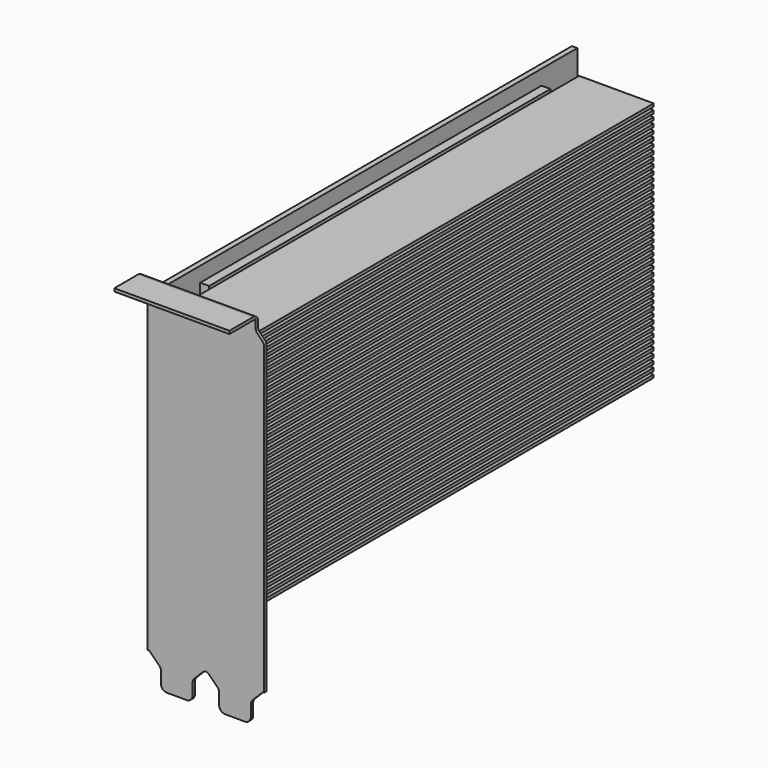
from build123d import *

# Parameters (mm, degrees)
F1_DEPTH    = 1
F2_SIZE     = 4
F0_W        = 38.5976333921
F0_H        = 1
F3_DEPTH    = 12
F4_T1_DEPTH = 1
F4_T3_DEPTH = 48.5976333921
F4_T5_DEPTH = 5.1421356237
F4_T7_DEPTH = 11
F5_W        = 1.8030845018
F5_H        = 92
F6_DEPTH    = 173
F7_W        = 143
F7_H        = 82
F8_DEPTH    = 3
F9_W        = 170
F9_H        = 1
F10_DEPTH   = 25


# Not quite as in the source:
# - a fillet or chamfer that OpenCascade refuses, or shapes differently, is made with other operations: its cross-section is extruded or revolved along the edge and cut away or added


with BuildPart() as f1:
    # F0 (on Front) → F1 (new body)
    with BuildSketch(Plane.XZ):
        Polygon((7.7390509516, 91.1776412405), (10.1390509516, 88.7776412405), (10.1390509516, -14.2223587595), (14.5890509516, -14.2223587595), (14.5890509516, -24.8223587595), (25.1890509516, -24.8223587595), (25.1890509516, -14.2223587595), (29.6390509516, -14.2223587595), (34.0890509516, -14.2223587595), (34.0890509516, -24.8223587595), (44.6890509516, -24.8223587595), (44.6890509516, -14.2223587595), (49.1390509516, -14.2223587595), (49.1390509516, 88.7776412405), (46.3366843437, 91.5800078484), (46.3366843437, 95.1776412405), (7.7390509516, 95.1776412405), align=None)
    extrude(amount=F1_DEPTH)

    # F2
    f2_edges = [f1.edges().sort_by_distance(p)[0] for p in [
        (14.589051, -0.5, -14.222359),
        (25.189051, -0.5, -14.222359),
        (34.089051, -0.5, -14.222359),
        (44.689051, -0.5, -14.222359),
    ]]
    chamfer(f2_edges, length=F2_SIZE)

    # F0 (on Front) → F3 (join)
    with BuildSketch(Plane.XZ):
        with Locations((27.0378676476, 95.6776412405)):
            Rectangle(F0_W, F0_H)
    extrude(amount=F3_DEPTH)

    # F4: fillet of radius 2 on 15 edges, made by hand

    # F4_s2 → F4_t1 (join)
    with BuildSketch(Plane.XZ):
        with BuildLine():
            ThreePointArc((46.3366843437, 92.4084349732), (46.4889252787, 91.6430681084), (46.9224707813, 90.9942214108))
            Line((46.9224707813, 90.9942214108), (46.3366843437, 91.5800078484))
            Line((46.3366843437, 91.5800078484), (46.3366843437, 92.4084349732))
        make_face()
        with BuildLine():
            ThreePointArc((10.1390509516, 87.9492141158), (9.9868100166, 88.7145809805), (9.553264514, 89.3634276781))
            Line((9.553264514, 89.3634276781), (10.1390509516, 88.7776412405))
            Line((10.1390509516, 88.7776412405), (10.1390509516, 87.9492141158))
        make_face()
        with BuildLine():
            ThreePointArc((14.003264514, -17.6365723219), (14.4368100166, -18.2854190195), (14.5890509516, -19.0507858842))
            Line((14.5890509516, -19.0507858842), (14.5890509516, -18.2223587595))
            Line((14.5890509516, -18.2223587595), (14.003264514, -17.6365723219))
        make_face()
        with BuildLine():
            ThreePointArc((25.1890509516, -19.0507858842), (25.3412918866, -18.2854190195), (25.7748373892, -17.6365723219))
            Line((25.7748373892, -17.6365723219), (25.1890509516, -18.2223587595))
            Line((25.1890509516, -18.2223587595), (25.1890509516, -19.0507858842))
        make_face()
        with BuildLine():
            ThreePointArc((28.603264514, -14.8081451971), (29.2521112116, -14.3745996945), (30.0174780763, -14.2223587595))
            Line((30.0174780763, -14.2223587595), (29.1890509516, -14.2223587595))
            Line((29.1890509516, -14.2223587595), (28.603264514, -14.8081451971))
        make_face()
        with BuildLine():
            ThreePointArc((29.2606238269, -14.2223587595), (30.0259906916, -14.3745996945), (30.6748373892, -14.8081451971))
            Line((30.6748373892, -14.8081451971), (30.0890509516, -14.2223587595))
            Line((30.0890509516, -14.2223587595), (29.2606238269, -14.2223587595))
        make_face()
        with BuildLine():
            ThreePointArc((33.503264514, -17.6365723219), (33.9368100166, -18.2854190195), (34.0890509516, -19.0507858842))
            Line((34.0890509516, -19.0507858842), (34.0890509516, -18.2223587595))
            Line((34.0890509516, -18.2223587595), (33.503264514, -17.6365723219))
        make_face()
        with BuildLine():
            ThreePointArc((44.6890509516, -19.0507858842), (44.8412918866, -18.2854190195), (45.2748373892, -17.6365723219))
            Line((45.2748373892, -17.6365723219), (44.6890509516, -18.2223587595))
            Line((44.6890509516, -18.2223587595), (44.6890509516, -19.0507858842))
        make_face()
    extrude(amount=F4_T1_DEPTH)

    # F4_s4 → F4_t3 (cut)
    with BuildSketch(Plane.YZ.offset(2.7390509516)):
        with BuildLine():
            ThreePointArc((0, 94.1776412405), (-0.5857864376, 95.5918548029), (-2, 96.1776412405))
            Line((-2, 96.1776412405), (0, 96.1776412405))
            Line((0, 96.1776412405), (0, 94.1776412405))
        make_face()
    extrude(amount=F4_T3_DEPTH, mode=Mode.SUBTRACT)

    # F4_s6 → F4_t5 (cut)
    with BuildSketch(Plane.XZ.offset(-2.0710678119)):
        with BuildLine():
            ThreePointArc((7.7390509516, 92.0060683653), (7.8912918866, 91.2407015005), (8.3248373892, 90.5918548029))
            Line((8.3248373892, 90.5918548029), (7.7390509516, 91.1776412405))
            Line((7.7390509516, 91.1776412405), (7.7390509516, 92.0060683653))
        make_face()
        with BuildLine():
            ThreePointArc((49.1390509516, 87.9492141158), (48.9868100166, 88.7145809805), (48.553264514, 89.3634276781))
            Line((48.553264514, 89.3634276781), (49.1390509516, 88.7776412405))
            Line((49.1390509516, 88.7776412405), (49.1390509516, 87.9492141158))
        make_face()
    extrude(amount=F4_T5_DEPTH, mode=Mode.SUBTRACT)

    # F4_s8 → F4_t7 (cut)
    with BuildSketch(Plane.XZ.offset(-5)):
        with BuildLine():
            ThreePointArc((14.5890509516, -22.8223587595), (15.1748373892, -24.2365723219), (16.5890509516, -24.8223587595))
            Line((16.5890509516, -24.8223587595), (14.5890509516, -24.8223587595))
            Line((14.5890509516, -24.8223587595), (14.5890509516, -22.8223587595))
        make_face()
        with BuildLine():
            ThreePointArc((23.1890509516, -24.8223587595), (24.603264514, -24.2365723219), (25.1890509516, -22.8223587595))
            Line((25.1890509516, -22.8223587595), (25.1890509516, -24.8223587595))
            Line((25.1890509516, -24.8223587595), (23.1890509516, -24.8223587595))
        make_face()
        with BuildLine():
            ThreePointArc((36.0890509516, -24.8223587595), (34.6748373892, -24.2365723219), (34.0890509516, -22.8223587595))
            Line((34.0890509516, -22.8223587595), (34.0890509516, -24.8223587595))
            Line((34.0890509516, -24.8223587595), (36.0890509516, -24.8223587595))
        make_face()
        with BuildLine():
            ThreePointArc((44.6890509516, -22.8223587595), (44.103264514, -24.2365723219), (42.6890509516, -24.8223587595))
            Line((42.6890509516, -24.8223587595), (44.6890509516, -24.8223587595))
            Line((44.6890509516, -24.8223587595), (44.6890509516, -22.8223587595))
        make_face()
    extrude(amount=F4_T7_DEPTH, mode=Mode.SUBTRACT)

    # F5 (on face) → F6 (join)
    with BuildSketch(Plane(origin=(0, 0, 0), x_dir=(-1, 0, 0), z_dir=(0, 1, 0))):
        with Locations((-14.0405932025, 48.1776412405)):
            Rectangle(F5_W, F5_H)
    extrude(amount=F6_DEPTH)

    # F7 (on face) → F8 (join)
    with BuildSketch(Plane.YZ.offset(14.9421354534)):
        with Locations((86.5, 48.1776412405)):
            Rectangle(F7_W, F7_H)
    extrude(amount=F8_DEPTH)

    # F9 (on face) → F10 (join)
    with BuildSketch(Plane.YZ.offset(17.9421354534)):
        with Locations((85, 7.6776412405)):
            Rectangle(F9_W, F9_H)
        with Locations((85, 9.6776412405)):
            Rectangle(F9_W, F9_H)
        with Locations((85, 11.6776412405)):
            Rectangle(F9_W, F9_H)
        with Locations((85, 13.6776412405)):
            Rectangle(F9_W, F9_H)
        with Locations((85, 15.6776412405)):
            Rectangle(F9_W, F9_H)
        with Locations((85, 17.6776412405)):
            Rectangle(F9_W, F9_H)
        with Locations((85, 19.6776412405)):
            Rectangle(F9_W, F9_H)
        with Locations((85, 21.6776412405)):
            Rectangle(F9_W, F9_H)
        with Locations((85, 23.6776412405)):
            Rectangle(F9_W, F9_H)
        with Locations((85, 25.6776412405)):
            Rectangle(F9_W, F9_H)
        with Locations((85, 27.6776412405)):
            Rectangle(F9_W, F9_H)
        with Locations((85, 29.6776412405)):
            Rectangle(F9_W, F9_H)
        with Locations((85, 31.6776412405)):
            Rectangle(F9_W, F9_H)
        with Locations((85, 33.6776412405)):
            Rectangle(F9_W, F9_H)
        with Locations((85, 35.6776412405)):
            Rectangle(F9_W, F9_H)
        with Locations((85, 37.6776412405)):
            Rectangle(F9_W, F9_H)
        with Locations((85, 39.6776412405)):
            Rectangle(F9_W, F9_H)
        with Locations((85, 41.6776412405)):
            Rectangle(F9_W, F9_H)
        with Locations((85, 43.6776412405)):
            Rectangle(F9_W, F9_H)
        with Locations((85, 45.6776412405)):
            Rectangle(F9_W, F9_H)
        with Locations((85, 47.6776412405)):
            Rectangle(F9_W, F9_H)
        with Locations((85, 49.6776412405)):
            Rectangle(F9_W, F9_H)
        with Locations((85, 51.6776412405)):
            Rectangle(F9_W, F9_H)
        with Locations((85, 53.6776412405)):
            Rectangle(F9_W, F9_H)
        with Locations((85, 55.6776412405)):
            Rectangle(F9_W, F9_H)
        with Locations((85, 57.6776412405)):
            Rectangle(F9_W, F9_H)
        with Locations((85, 59.6776412405)):
            Rectangle(F9_W, F9_H)
        with Locations((85, 61.6776412405)):
            Rectangle(F9_W, F9_H)
        with Locations((85, 63.6776412405)):
            Rectangle(F9_W, F9_H)
        with Locations((85, 65.6776412405)):
            Rectangle(F9_W, F9_H)
        with Locations((85, 67.6776412405)):
            Rectangle(F9_W, F9_H)
        with Locations((85, 69.6776412405)):
            Rectangle(F9_W, F9_H)
        with Locations((85, 71.6776412405)):
            Rectangle(F9_W, F9_H)
        with Locations((85, 73.6776412405)):
            Rectangle(F9_W, F9_H)
        with Locations((85, 75.6776412405)):
            Rectangle(F9_W, F9_H)
        with Locations((85, 77.6776412405)):
            Rectangle(F9_W, F9_H)
        with Locations((85, 79.6776412405)):
            Rectangle(F9_W, F9_H)
        with Locations((85, 81.6776412405)):
            Rectangle(F9_W, F9_H)
        with Locations((85, 83.6776412405)):
            Rectangle(F9_W, F9_H)
        with Locations((85, 85.6776412405)):
            Rectangle(F9_W, F9_H)
        with Locations((85, 87.6776412405)):
            Rectangle(F9_W, F9_H)
    extrude(amount=F10_DEPTH)


solid = f1.part
